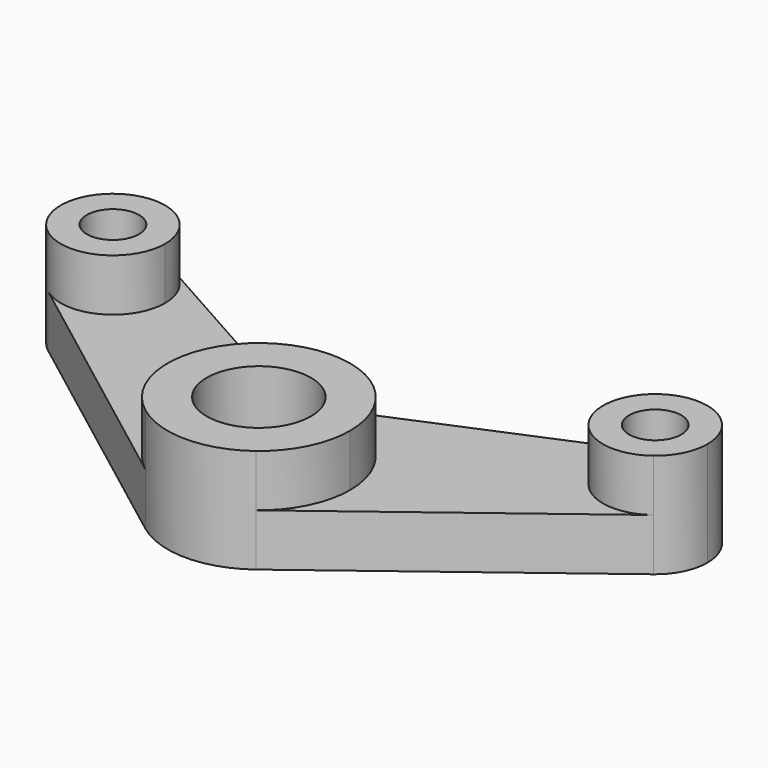
from build123d import *

# Parameters (mm, degrees)
F0_R     = 1
F1_DEPTH = 2
F0_R_2   = 0.5
F2_DEPTH = 1
F3_DEPTH = 2
F4_DEPTH = 1


with BuildPart() as f1:
    # F0 (on Top) → F1 (new body)
    with BuildSketch(Plane.XY):
        with BuildLine():
            ThreePointArc((1.057580206, -1.3942826499), (1.5673648842, -0.7783747939), (1.75, 0))
            ThreePointArc((1.75, 0), (0.9681904098, 1.4577747873), (-0.6786940919, 1.6130326499))
            ThreePointArc((-0.6786940919, 1.6130326499), (-1.7362742979, 0.21875), (-1.057580206, -1.3942826499))
            ThreePointArc((-1.057580206, -1.3942826499), (0, -1.75), (1.057580206, -1.3942826499))
        make_face()
        Circle(F0_R, mode=Mode.SUBTRACT)
    extrude(amount=F1_DEPTH)



with BuildPart() as f1b:
    # F0 (on Top) → F1, piece 2 (new body)
    with BuildSketch(Plane.XY):
        with BuildLine():
            ThreePointArc((6.1961524227, 3), (5.7494040854, 3.8330141642), (4.8083272274, 3.9217329428))
            ThreePointArc((4.8083272274, 3.9217329428), (4.3301270189, 2.5), (5.800483969, 2.2032670572))
            ThreePointArc((5.800483969, 2.2032670572), (6.0917894994, 2.5552144035), (6.1961524227, 3))
        make_face()
        with Locations((5.1961524227, 3)):
            Circle(F0_R_2, mode=Mode.SUBTRACT)
    extrude(amount=F1_DEPTH)


with BuildPart() as f1_1:
    add(f1.part)

    add(f1b.part)  # F2 merges F1b
    # F0 (on Top) → F2 (join)
    with BuildSketch(Plane.XY):
        with BuildLine():
            ThreePointArc((-0.6786940919, 1.6130326499), (0.9681904098, 1.4577747873), (1.75, 0))
            ThreePointArc((1.75, 0), (1.5673648842, -0.7783747939), (1.057580206, -1.3942826499))
            Line((1.057580206, -1.3942826499), (5.800483969, 2.2032670572))
            ThreePointArc((5.800483969, 2.2032670572), (4.3301270189, 2.5), (4.8083272274, 3.9217329428))
            Line((4.8083272274, 3.9217329428), (-0.6786940919, 1.6130326499))
        make_face()
    extrude(amount=F2_DEPTH)


with BuildPart() as f3:
    # F0 (on Top) → F3 (new body)
    with BuildSketch(Plane.XY):
        with BuildLine():
            ThreePointArc((-4.1961524227, 3), (-4.3332649527, 3.5053960962), (-4.7070028508, 3.8721999176))
            ThreePointArc((-4.7070028508, 3.8721999176), (-6.032603823, 3.5480411071), (-5.800483969, 2.2032670572))
            ThreePointArc((-5.800483969, 2.2032670572), (-4.7513668262, 2.1043629233), (-4.1961524227, 3))
        make_face()
        with Locations((-5.1961524227, 3)):
            Circle(F0_R_2, mode=Mode.SUBTRACT)
    extrude(amount=F3_DEPTH)

    # F0 (on Top) → F4 (join)
    with BuildSketch(Plane.XY):
        with BuildLine():
            ThreePointArc((-1.057580206, -1.3942826499), (-1.7362742979, 0.21875), (-0.6786940919, 1.6130326499))
            Line((-0.6786940919, 1.6130326499), (-4.7070028508, 3.8721999176))
            ThreePointArc((-4.7070028508, 3.8721999176), (-4.3332649527, 3.5053960962), (-4.1961524227, 3))
            ThreePointArc((-4.1961524227, 3), (-4.7513668262, 2.1043629233), (-5.800483969, 2.2032670572))
            Line((-5.800483969, 2.2032670572), (-1.057580206, -1.3942826499))
        make_face()
    extrude(amount=F4_DEPTH)


solid = Compound([f1_1.part, f3.part])
